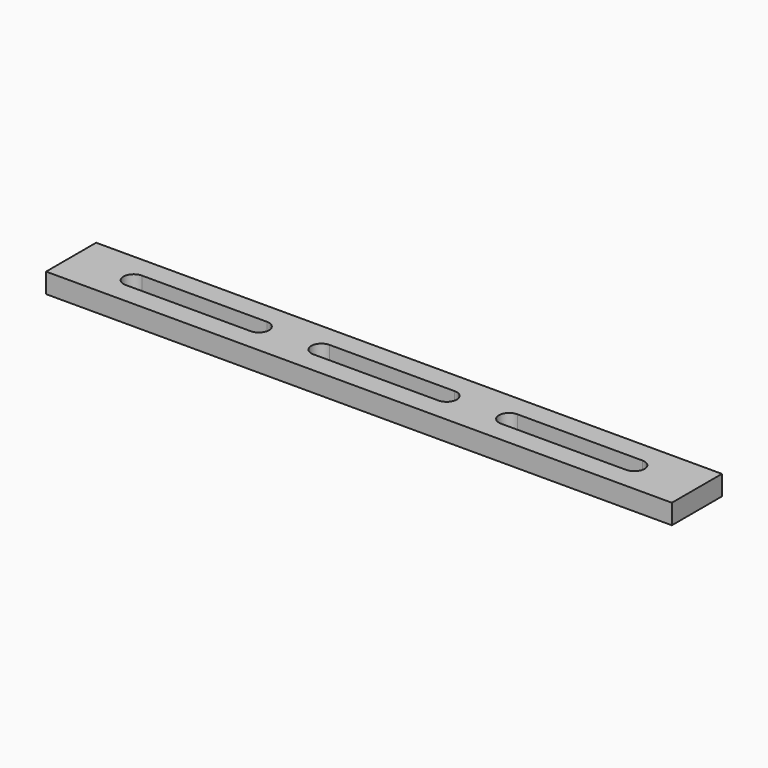
from build123d import *

# Parameters (mm, degrees)
F0_W     = 200
F0_H     = 20
F1_DEPTH = 6.35


# Not quite as in the source:
# - a length typed as a fraction of an inch, garbled in the dataset ("3 / 203.2 mm" for 3/8 in), is restored


with BuildPart() as f1:
    # F0 (on Top) → F1 (new body)
    with BuildSketch(Plane.XY):
        Rectangle(F0_W, F0_H)
        with BuildLine():
            Line((-80, 3.25), (-40, 3.25))
            ThreePointArc((-40, 3.25), (-36.75, 0), (-40, -3.25))
            Line((-40, -3.25), (-80, -3.25))
            ThreePointArc((-80, -3.25), (-83.25, 0), (-80, 3.25))
        make_face(mode=Mode.SUBTRACT)
        with BuildLine():
            Line((-20, 3.25), (20, 3.25))
            ThreePointArc((20, 3.25), (23.25, 0), (20, -3.25))
            Line((20, -3.25), (-20, -3.25))
            ThreePointArc((-20, -3.25), (-23.25, 0), (-20, 3.25))
        make_face(mode=Mode.SUBTRACT)
        with BuildLine():
            Line((80, -3.25), (40, -3.25))
            ThreePointArc((40, -3.25), (36.75, 0), (40, 3.25))
            Line((40, 3.25), (80, 3.25))
            ThreePointArc((80, 3.25), (83.25, 0), (80, -3.25))
        make_face(mode=Mode.SUBTRACT)
    extrude(amount=F1_DEPTH)


solid = f1.part
